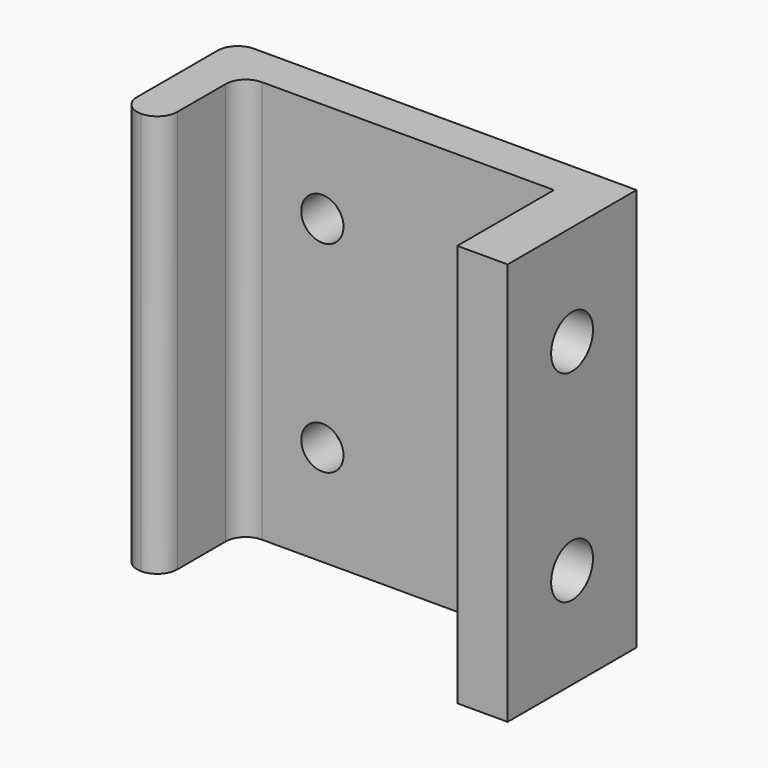
from build123d import *

# Parameters (mm, degrees)
F0_W     = 4
F0_H     = 10
F0_W_2   = 5
F0_H_2   = 12
F1_DEPTH = 40
F3_R     = 1.99999
F4_D     = 5.2
F4_DEPTH = 12
F4_TIP   = 1.5622376095
F6_D     = 4.2
F6_DEPTH = 12
F6_TIP   = 1.2618073


# Not quite as in the source:
# - a fillet or chamfer is up to 0.001 mm smaller than in the source, because OpenCascade refuses the exact size


with BuildPart() as f1:
    # F0 (on Top) → F1 (new body)
    with BuildSketch(Plane.XY):
        Polygon((-36.5682695345, 36.2048765272), (-76.5682695345, 36.2048765272), (-76.5682695345, 32.2048765272), (-72.5682695345, 32.2048765272), (-41.5682695345, 32.2048765272), (-36.5682695345, 32.2048765272), align=None)
        with Locations((-74.5682695345, 27.2048765272)):
            Rectangle(F0_W, F0_H)
        with Locations((-39.0682695345, 26.2048765272)):
            Rectangle(F0_W_2, F0_H_2)
    extrude(amount=F1_DEPTH)

    # F3 (radius 2 in the source; OpenCascade refuses exactly that, so slightly less here)
    f3_edges = [f1.edges().sort_by_distance(p)[0] for p in [
        (-76.56827, 36.204877, 20),
        (-72.56827, 32.204877, 20),
        (-76.56827, 22.204877, 20),
        (-72.56827, 22.204877, 20),
    ]]
    fillet(f3_edges, radius=F3_R)

    # F4
    with Locations(Plane.YZ.offset(-36.5682695345)):
        with Locations((28.2048765272, 10), (28.2048765272, 30)):
            Hole(F4_D / 2, depth=F4_DEPTH)
            with Locations((0, 0, -(F4_DEPTH + F4_TIP / 2))):  # 118° drill point
                Cone(0, F4_D / 2, F4_TIP, mode=Mode.SUBTRACT)

    # F6
    with Locations(Plane(origin=(0, 36.2048765272, 0), x_dir=(-1, 0, 0), z_dir=(0, 1, 0))):
        with Locations((64.5682695345, 10), (64.5682695345, 30)):
            Hole(F6_D / 2, depth=F6_DEPTH)
            with Locations((0, 0, -(F6_DEPTH + F6_TIP / 2))):  # 118° drill point
                Cone(0, F6_D / 2, F6_TIP, mode=Mode.SUBTRACT)


solid = f1.part
